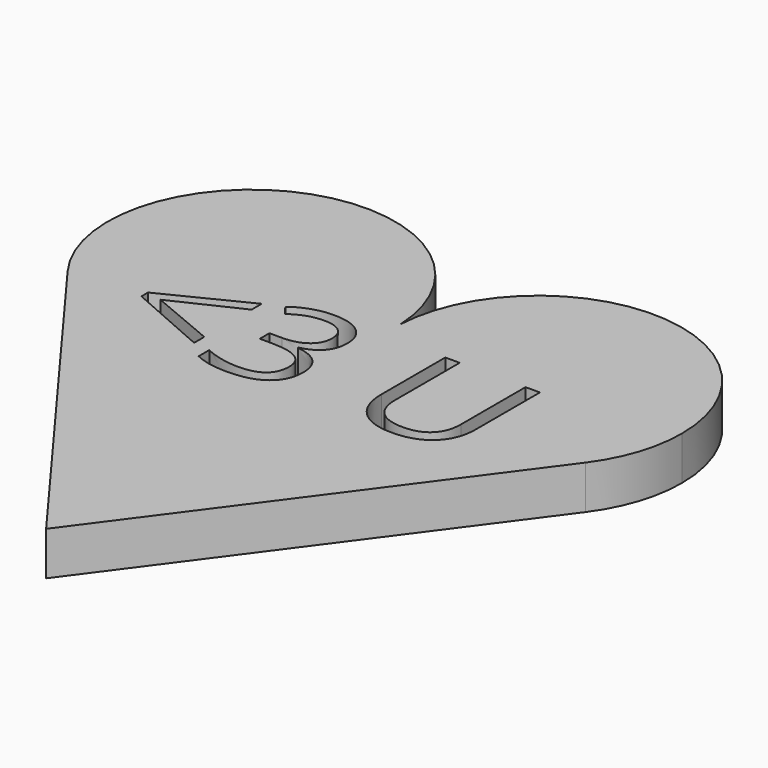
from build123d import *

# Parameters (mm, degrees)
F1_DEPTH     = 2.54
F2_TEXT_SIZE = 10.0898375321
F3_DEPTH     = 25.4


# Not quite as in the source:
# - Text() gives the source's letters only with a copy of the font that has no kerning and outlines rounded to 1/6400 em; it was checked with that copy


with BuildPart() as f1:
    # F0 (on Top) → F1 (new body)
    with BuildSketch(Plane.XY):
        with BuildLine():
            ThreePointArc((0, 24.9864145082), (5.9402844739, 17.3912160404), (15.0909087391, 20.4309684897))
            ThreePointArc((15.0909087391, 20.4309684897), (16.3083493995, 22.7858839577), (16.7282046217, 25.4034229193))
            ThreePointArc((16.7282046217, 25.4034229193), (8.5674736024, 33.7701236711), (0, 25.8204313303))
            ThreePointArc((0, 25.8204313303), (0.0077961301, 25.6119918999), (0.0103953783, 25.4034229193))
            ThreePointArc((0.0103953783, 25.4034229193), (0.0077961301, 25.1948539386), (0, 24.9864145082))
        make_face()
        with BuildLine():
            Line((0, 0), (15.0909087391, 20.4309684897))
            ThreePointArc((15.0909087391, 20.4309684897), (5.9402844739, 17.3912160404), (0, 24.9864145082))
            ThreePointArc((0, 24.9864145082), (-5.9402844739, 17.3912160404), (-15.0909087391, 20.4309684897))
            Line((-15.0909087391, 20.4309684897), (0, 0))
        make_face()
        with BuildLine():
            ThreePointArc((-15.0909087391, 20.4309684897), (-5.9402844739, 17.3912160404), (0, 24.9864145082))
            ThreePointArc((0, 24.9864145082), (-0.0103953783, 25.4034229193), (0, 25.8204313303))
            ThreePointArc((0, 25.8204313303), (-11.1737365422, 33.2851678878), (-15.0909087391, 20.4309684897))
        make_face()
        with BuildLine():
            ThreePointArc((0, 25.8204313303), (-0.0103953783, 25.4034229193), (0, 24.9864145082))
            ThreePointArc((0, 24.9864145082), (0.0077961301, 25.1948539386), (0.0103953783, 25.4034229193))
            ThreePointArc((0.0103953783, 25.4034229193), (0.0077961301, 25.6119918999), (0, 25.8204313303))
        make_face()
    extrude(amount=F1_DEPTH)

    # F2 (on face) → F3 (cut)
    with BuildSketch(Plane.XY.offset(2.54)):
        with Locations((-11.4372260869, 17.3279065639)):
            Text('<3 U', F2_TEXT_SIZE, font='Open Sans', text_align=(TextAlign.LEFT, TextAlign.BOTTOM))
    extrude(amount=-F3_DEPTH, mode=Mode.SUBTRACT)


solid = f1.part
